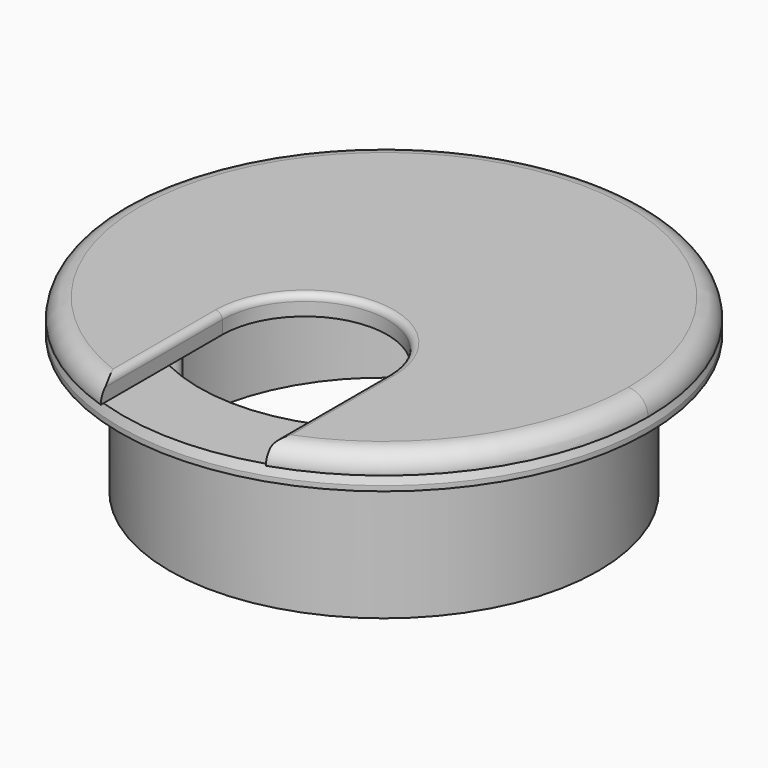
from build123d import *

# Parameters (mm, degrees)
F0_R        = 30.48
F0_R_2      = 20.955
F1_DEPTH    = 1.6002
F2_R        = 24.765
F2_R_2      = 22.225
F3_DEPTH    = 15.875
F5_DEPTH    = 2.286
F6_R        = 2.28599
F7_DEPTH    = 2.287
F8_T1_DEPTH = 17.0113255723
F8_T4_ANGLE = 180
F10_DEPTH   = 3.937
F11_SIZE2   = 1.016
F11_SIZE    = 0.381
F12_SIZE2   = 0.381
F12_SIZE    = 1.016


# Not quite as in the source:
# - a fillet or chamfer that OpenCascade refuses, or shapes differently, is made with other operations: its cross-section is extruded or revolved along the edge and cut away or added
# - a fillet or chamfer is up to 0.001 mm smaller than in the source, because OpenCascade refuses the exact size


with BuildPart() as f1:
    # F0 (on Top) → F1 (new body)
    with BuildSketch(Plane.XY):
        Circle(F0_R)
        Circle(F0_R_2, mode=Mode.SUBTRACT)
    extrude(amount=-F1_DEPTH)

    # F2 (on face) → F3 (join)
    with BuildSketch(Plane(origin=(0, 0, -1.6002), x_dir=(1, 0, 0), z_dir=(0, 0, -1))):
        Circle(F2_R)
        Circle(F2_R_2, mode=Mode.SUBTRACT)
    extrude(amount=F3_DEPTH)

    # F11
    f11_edges = [f1.edges().sort_by_distance(p)[0] for p in [
        (-30.48, 0, 0),
    ]]
    f11_side = f1.faces().sort_by_distance((-29.617895, 0, 0))[0]
    chamfer(f11_edges, length=F11_SIZE, length2=F11_SIZE2, reference=f11_side)

    # F12
    f12_edges = [f1.edges().sort_by_distance(p)[0] for p in [
        (-20.955, 0, 0),
    ]]
    f12_side = f1.faces().sort_by_distance((-20.955, 0, -0.8001))[0]
    chamfer(f12_edges, length=F12_SIZE, length2=F12_SIZE2, reference=f12_side)


with BuildPart() as f5:
    # F4 (on face) → F5 (new body)
    with BuildSketch(Plane.XY):
        with BuildLine():
            Line((-9.525, -18.66511184), (-9.525, -28.9534933126))
            ThreePointArc((-9.525, -28.9534933126), (0, -30.48), (9.525, -28.9534933126))
            Line((9.525, -28.9534933126), (9.525, -18.66511184))
            ThreePointArc((9.525, -18.66511184), (0, -20.955), (-9.525, -18.66511184))
        make_face()
        with BuildLine():
            ThreePointArc((9.525, -28.9534933126), (24.6916220609, -17.8704840449), (30.48, 0))
            ThreePointArc((30.48, 0), (-17.8704840449, 24.6916220609), (-9.525, -28.9534933126))
            Line((-9.525, -28.9534933126), (-9.525, -18.66511184))
            ThreePointArc((-9.525, -18.66511184), (-10.9433918417, 17.8704840449), (20.955, 0))
            ThreePointArc((20.955, 0), (17.8704840449, -10.9433918417), (9.525, -18.66511184))
            Line((9.525, -18.66511184), (9.525, -28.9534933126))
        make_face()
        with BuildLine():
            Line((-9.525, -11.43), (-9.525, -18.66511184))
            ThreePointArc((-9.525, -18.66511184), (0, -20.955), (9.525, -18.66511184))
            Line((9.525, -18.66511184), (9.525, -11.43))
            ThreePointArc((9.525, -11.43), (0, -1.905), (-9.525, -11.43))
        make_face()
        with BuildLine():
            ThreePointArc((20.955, 0), (-10.9433918417, 17.8704840449), (-9.525, -18.66511184))
            Line((-9.525, -18.66511184), (-9.525, -11.43))
            ThreePointArc((-9.525, -11.43), (0, -1.905), (9.525, -11.43))
            Line((9.525, -11.43), (9.525, -18.66511184))
            ThreePointArc((9.525, -18.66511184), (17.8704840449, -10.9433918417), (20.955, 0))
        make_face()
    extrude(amount=F5_DEPTH)

    # F6 (radius 2.286 in the source; OpenCascade refuses exactly that, so slightly less here)
    f6_edges = [f5.edges().sort_by_distance(p)[0] for p in [
        (-9.525, 28.953493, 2.286),
    ]]
    fillet(f6_edges, radius=F6_R)

    # F4 (on face) → F7 (cut, through all)
    with BuildSketch(Plane.XY):
        with BuildLine():
            Line((-9.525, -11.43), (-9.525, -18.66511184))
            ThreePointArc((-9.525, -18.66511184), (0, -20.955), (9.525, -18.66511184))
            Line((9.525, -18.66511184), (9.525, -11.43))
            ThreePointArc((9.525, -11.43), (0, -1.905), (-9.525, -11.43))
        make_face()
        with BuildLine():
            Line((-9.525, -18.66511184), (-9.525, -28.9534933126))
            ThreePointArc((-9.525, -28.9534933126), (0, -30.48), (9.525, -28.9534933126))
            Line((9.525, -28.9534933126), (9.525, -18.66511184))
            ThreePointArc((9.525, -18.66511184), (0, -20.955), (-9.525, -18.66511184))
        make_face()
    extrude(amount=F7_DEPTH, mode=Mode.SUBTRACT)

    # F8: fillet of radius 0.762 on 3 edges, made by hand

    # F8_s2 → F8_t1 (cut)
    with BuildSketch(Plane.XZ.offset(11.43)):
        with BuildLine():
            ThreePointArc((-9.525, 1.524), (-9.7481846327, 2.0628153673), (-10.287, 2.286))
            Line((-10.287, 2.286), (-9.525, 2.286))
            Line((-9.525, 2.286), (-9.525, 1.524))
        make_face()
        with BuildLine():
            ThreePointArc((9.525, 1.524), (9.7481846327, 2.0628153673), (10.287, 2.286))
            Line((10.287, 2.286), (9.525, 2.286))
            Line((9.525, 2.286), (9.525, 1.524))
        make_face()
    extrude(amount=F8_T1_DEPTH, mode=Mode.SUBTRACT)

    # F8_s3 → F8_t4 (revolve, cut)
    with BuildSketch(Plane.XZ.offset(11.43)):
        with BuildLine():
            ThreePointArc((-9.525, 1.524), (-9.7481846327, 2.0628153673), (-10.287, 2.286))
            Line((-10.287, 2.286), (-9.525, 2.286))
            Line((-9.525, 2.286), (-9.525, 1.524))
        make_face()
    revolve(axis=Axis((0, -11.43, 2.286), (0, 0, -1)), revolution_arc=F8_T4_ANGLE, mode=Mode.SUBTRACT)

    # F9 (on face) → F10 (join)
    with BuildSketch(Plane(origin=(0, 0, 0), x_dir=(1, 0, 0), z_dir=(0, 0, -1))):
        with BuildLine():
            ThreePointArc((-12.4545810811, 16.6939807744), (0, -20.828), (12.4545810811, 16.6939807744))
            ThreePointArc((12.4545810811, 16.6939807744), (11.032700015, 16.4871807893), (11.2395, 15.0652997232))
            ThreePointArc((11.2395, 15.0652997232), (0, -18.796), (-11.2395, 15.0652997232))
            ThreePointArc((-11.2395, 15.0652997232), (-11.032700015, 16.4871807893), (-12.4545810811, 16.6939807744))
        make_face()
    extrude(amount=F10_DEPTH)


solid = Compound([f1.part, f5.part])
